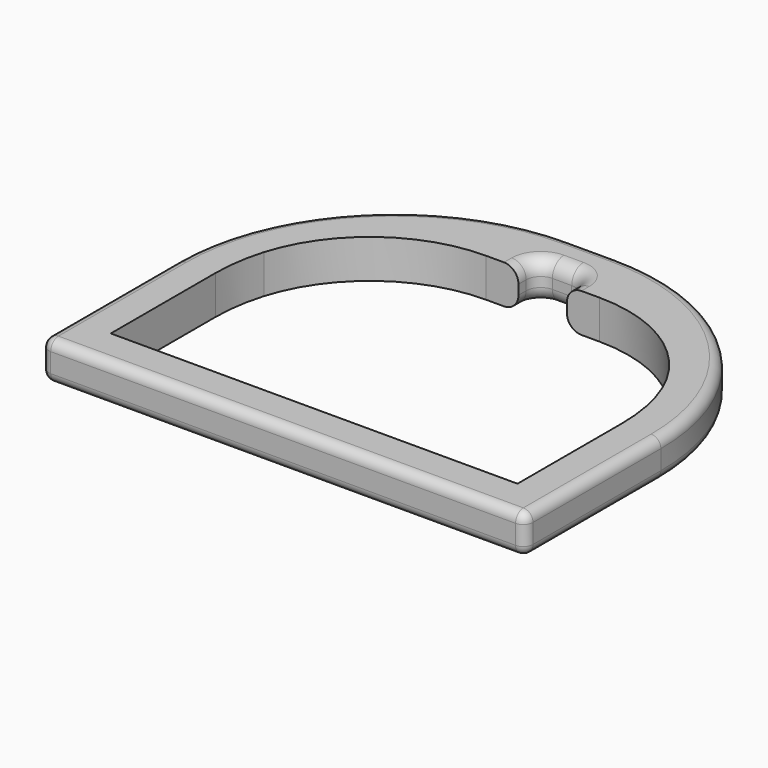
from build123d import *

# Parameters (mm, degrees)
F1_DEPTH = 8
F2_R     = 2
F3_F1_R  = 3
F3_F2_R  = 3


with BuildPart() as f1:
    # F0 (on Top) → F1 (new body)
    with BuildSketch(Plane.XY):
        with BuildLine():
            Line((55, 0), (45, 0))
            ThreePointArc((45, 0), (13.1801948466, -13.1801948466), (0, -45))
            Line((0, -45), (0, -80))
            Line((0, -80), (100, -80))
            Line((100, -80), (100, -45))
            ThreePointArc((100, -45), (86.8198051534, -13.1801948466), (55, 0))
        make_face()
        with BuildLine():
            Line((45, -13), (45, -8))
            Line((45, -8), (55, -8))
            Line((55, -8), (55, -13))
            Line((55, -13), (61.7082039325, -13))
            ThreePointArc((61.7082039325, -13), (79.6366330725, -18.9464882279), (90.4576493575, -34.4285714286))
            ThreePointArc((90.4576493575, -34.4285714286), (91.6123819645, -39.6583254605), (92, -45))
            Line((92, -45), (92, -72))
            Line((92, -72), (8, -72))
            Line((8, -72), (8, -45))
            ThreePointArc((8, -45), (8.3876180355, -39.6583254605), (9.5423506425, -34.4285714286))
            ThreePointArc((9.5423506425, -34.4285714286), (20.3633669275, -18.9464882279), (38.2917960675, -13))
            Line((38.2917960675, -13), (45, -13))
        make_face(mode=Mode.SUBTRACT)
    extrude(amount=F1_DEPTH)

    # F2
    f2_edges = [f1.edges().sort_by_distance(p)[0] for p in [
        (0, -80, 4),
        (100, -80, 4),
        (50, -80, 8),
        (0, -62.5, 8),
        (50, -80, 0),
        (86.819805, -13.180195, 0),
    ]]
    fillet(f2_edges, radius=F2_R)

    # F3: fillet of radius 3 on 4 edges, made by hand

    # F3_f1
    f3_f1_edges = [f1.edges().sort_by_distance(p)[0] for p in [
        (45, -8, 4),
        (55, -8, 4),
    ]]
    fillet(f3_f1_edges, radius=F3_F1_R)

    # F3_f2
    f3_f2_edges = [f1.edges().sort_by_distance(p)[0] for p in [
        (50, -8, 0),
        (50, -8, 8),
        (45.8786796564, -8.8786796564, 8),
        (54.1213203436, -8.8786796564, 8),
        (45.8786796564, -8.8786796564, 0),
        (54.1213203436, -8.8786796564, 0),
    ]]
    fillet(f3_f2_edges, radius=F3_F2_R)


solid = f1.part
